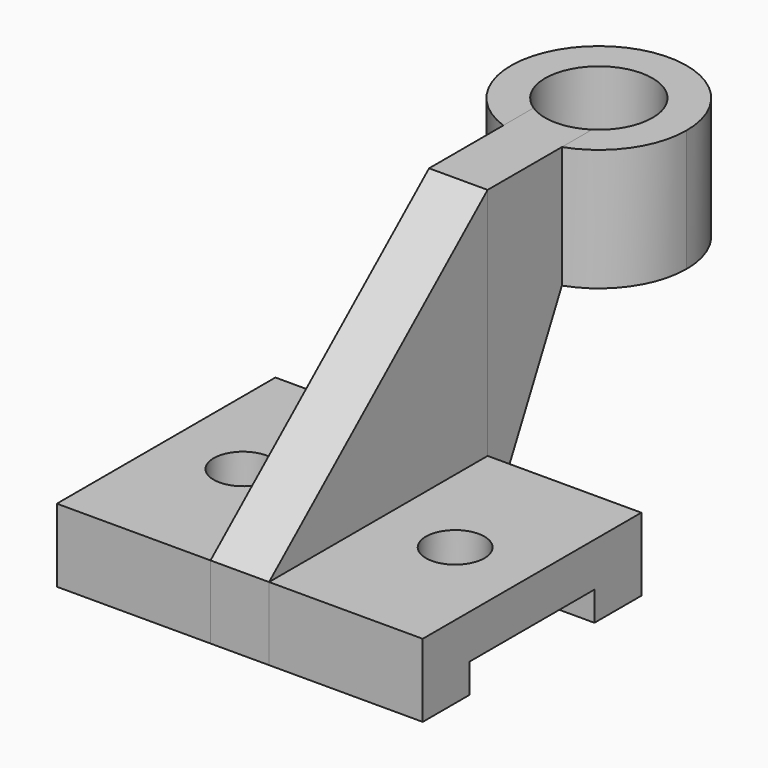
from build123d import *

# Parameters (mm, degrees)
F0_W      = 31.5
F0_H      = 56
F0_R      = 6
F1_DEPTH  = 15
F0_W_2    = 6
F2_DEPTH  = 63
F4_DEPTH  = 25
F5_DEPTH  = 36
F7_DEPTH  = 91.3
F8_DEPTH  = 25
F10_DEPTH = 25
F11_W     = 32
F11_H     = 6
F12_DEPTH = 107.5


with BuildPart() as f1:
    # F0 (on Top) → F1 (new body)
    with BuildSketch(Plane.XY):
        with Locations((-21.75, 0)):
            Rectangle(F0_W, F0_H)
        with Locations((-21.75, 0)):
            Circle(F0_R, mode=Mode.SUBTRACT)
    extrude(amount=F1_DEPTH)


with BuildPart() as f1b:
    # F0 (on Top) → F1, piece 2 (new body)
    with BuildSketch(Plane.XY):
        with Locations((21.75, 0)):
            Rectangle(F0_W, F0_H)
        with Locations((21.75, 0)):
            Circle(F0_R, mode=Mode.SUBTRACT)
    extrude(amount=F1_DEPTH)


with BuildPart() as f2:
    # F0 (on Top) → F2 (new body)
    with BuildSketch(Plane.XY):
        with Locations((3, 0)):
            Rectangle(F0_W_2, F0_H)
        with Locations((-3, 0)):
            Rectangle(F0_W_2, F0_H)
    extrude(amount=F2_DEPTH)

    # F3 (on face) → F4 (cut)
    with BuildSketch(Plane.YZ.offset(6)):
        Polygon((-28, 63), (-28, 15), (28, 63), align=None)
    extrude(amount=-F4_DEPTH, mode=Mode.SUBTRACT)


with BuildPart() as f5:
    # F5 (new): a face of the model
    f5_faces = [f2.part.faces().sort_by_distance(p)[0] for p in [
        (0, 28, 31.5),
    ]]
    extrude(f5_faces, amount=F5_DEPTH)

    # F6 (on face) → F7 (cut)
    with BuildSketch(Plane.XY.offset(63)):
        with BuildLine():
            Line((-6, 64), (-6, 54.7804555427))
            ThreePointArc((-6, 54.7804555427), (0, 53), (6, 54.7804555427))
            Line((6, 54.7804555427), (6, 64))
            Line((6, 64), (-6, 64))
        make_face()
    extrude(amount=-F7_DEPTH, mode=Mode.SUBTRACT)

    # F9 (on face) → F10 (cut)
    with BuildSketch(Plane.YZ.offset(6)):
        Polygon((47.0294372515, 38), (28, 0), (54.7804555427, 0), (54.7804555427, 38), align=None)
    extrude(amount=-F10_DEPTH, mode=Mode.SUBTRACT)


with BuildPart() as f8:
    # F6 (on face) → F8 (new body)
    with BuildSketch(Plane.XY.offset(63)):
        with BuildLine():
            ThreePointArc((-6, 54.7804555427), (-5.2440442409, 73.6695398029), (11, 64))
            ThreePointArc((11, 64), (9.6695398029, 58.7559557591), (6, 54.7804555427))
            Line((6, 54.7804555427), (6, 47.0294372515))
            ThreePointArc((6, 47.0294372515), (14.6969384567, 53.6076951546), (18, 64))
            ThreePointArc((18, 64), (-10.3923048454, 78.6969384567), (-6, 47.0294372515))
            Line((-6, 47.0294372515), (-6, 54.7804555427))
        make_face()
    extrude(amount=-F8_DEPTH)


with BuildPart() as f12_tool:
    # F11 (on face) → F12 (new body)
    with BuildSketch(Plane.YZ.offset(37.5)):
        with Locations((0, 3)):
            Rectangle(F11_W, F11_H)
    extrude(amount=-F12_DEPTH)


with BuildPart() as f1_1:
    add(f1.part)

    # F12: cut by f12_tool
    add(f12_tool.part, mode=Mode.SUBTRACT)


with BuildPart() as f1b_1:
    add(f1b.part)

    # F12: cut by f12_tool
    add(f12_tool.part, mode=Mode.SUBTRACT)


with BuildPart() as f2_1:
    add(f2.part)

    # F12: cut by f12_tool
    add(f12_tool.part, mode=Mode.SUBTRACT)


solid = Compound([f5.part, f8.part, f1_1.part, f1b_1.part, f2_1.part])
